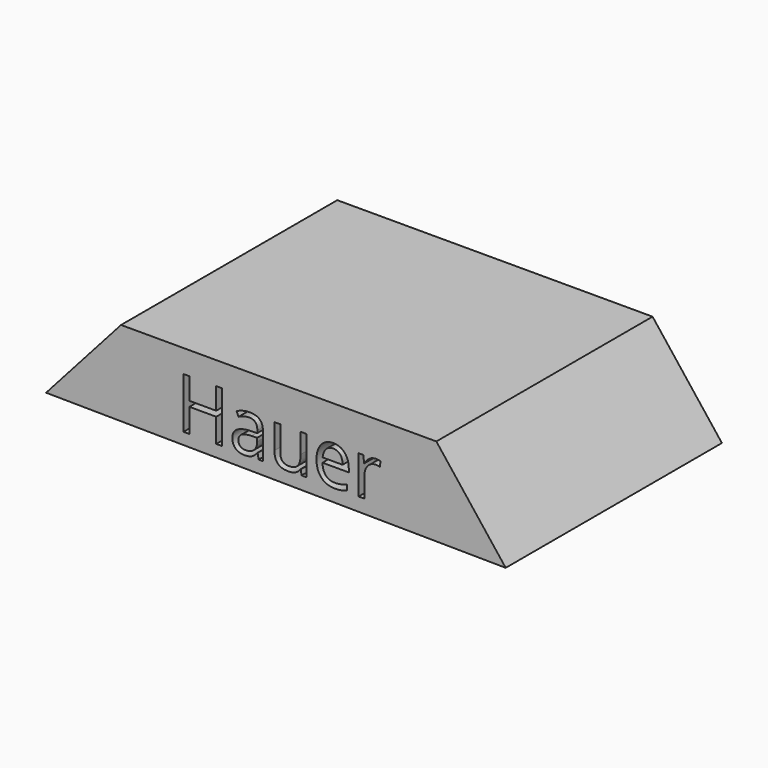
from build123d import *

# Parameters (mm, degrees)
F1_DEPTH     = 60.96
F2_TEXT_SIZE = 16.0801023917
F3_DEPTH     = 12.7


# Not quite as in the source:
# - Text() gives the source's letters only with a copy of the font that has no kerning and outlines rounded to 1/6400 em; it was checked with that copy


with BuildPart() as f1:
    # F0 (on Front) → F1 (new body)
    with BuildSketch(Plane.XZ):
        Polygon((35.56, 0), (0, 0), (-35.56, 0), (-52.4693827913, -18.9534369869), (51.2020461368, -20.0121561221), align=None)
    extrude(amount=F1_DEPTH)

    # F2 (on face) → F3 (cut)
    with BuildSketch(Plane.XZ.offset(60.96)):
        with Locations((-23.0519752949, -16.6429060046)):
            Text('Hauer', F2_TEXT_SIZE, font='Open Sans', text_align=(TextAlign.LEFT, TextAlign.BOTTOM))
    extrude(amount=-F3_DEPTH, mode=Mode.SUBTRACT)


solid = f1.part
